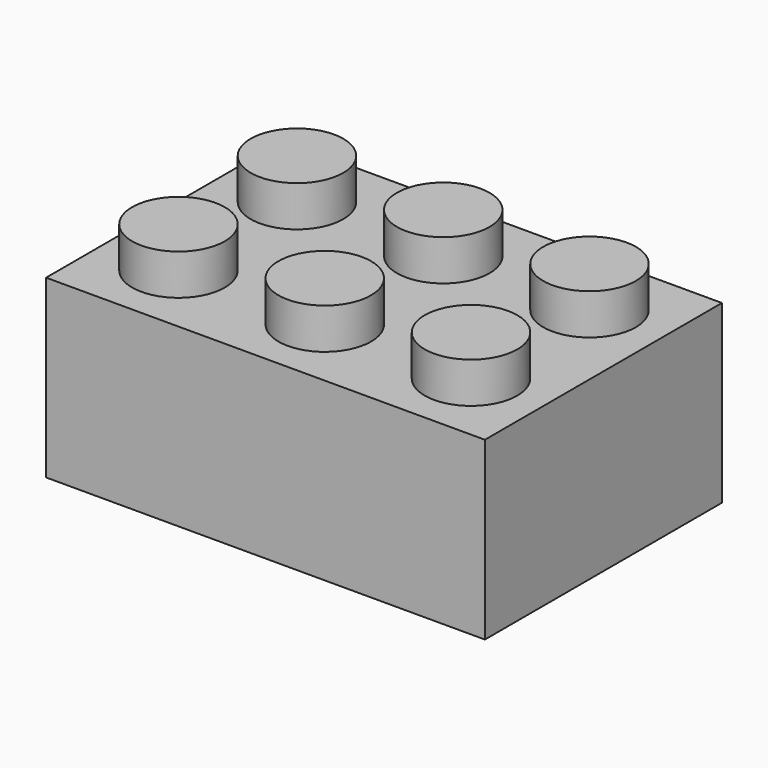
from build123d import *

# Parameters (mm, degrees)
F0_W        = 23.7
F0_H        = 8
F0_R        = 2.5
F1_DEPTH    = 9.5
F2_DEPTH    = 2.2
F4_T        = -1.5
F5_R        = 3
F6_DEPTH    = 7.9248
F7_T        = 1
F7_T3_DEPTH = 10
F7_T5_DEPTH = 15
F7_T7_DEPTH = 22.7


# Not quite as in the source:
# - a shell that OpenCascade refuses in one call is made with other operations: the cavity is built on its own and cut out


with BuildPart() as f1:
    # F0 (on Top) → F1 (new body)
    with BuildSketch(Plane.XY):
        with Locations((11.85, 4)):
            Rectangle(F0_W, F0_H)
        with Locations((3.95, 4)):
            Circle(F0_R, mode=Mode.SUBTRACT)
        with Locations((11.85, 4)):
            Circle(F0_R, mode=Mode.SUBTRACT)
        with Locations((19.75, 4)):
            Circle(F0_R, mode=Mode.SUBTRACT)
        with Locations((19.75, 4)):
            Circle(F0_R)
        with Locations((11.85, 4)):
            Circle(F0_R)
        with Locations((3.95, 4)):
            Circle(F0_R)
    extrude(amount=-F1_DEPTH)

    # F0 (on Top) → F2 (join)
    with BuildSketch(Plane.XY):
        with Locations((3.95, 4)):
            Circle(F0_R)
        with Locations((11.85, 4)):
            Circle(F0_R)
        with Locations((19.75, 4)):
            Circle(F0_R)
    extrude(amount=F2_DEPTH)

    # F3: F1 across face


with BuildPart() as f1_1:
    add(f1.part)
    add(f1.part.mirror(Plane(origin=(11.85, 0, -4.75), x_dir=(1, 0, 0), z_dir=(0, -1, 0))))

    # F4
    f4_openings = [f1_1.faces().sort_by_distance(p)[0] for p in [
        (11.85, 0, -9.5),
    ]]
    offset(amount=F4_T, openings=f4_openings, kind=Kind.INTERSECTION)

    # F5 (on face) → F6 (join)
    with BuildSketch(Plane(origin=(0, 0, -1.5), x_dir=(1, 0, 0), z_dir=(0, 0, -1))):
        with Locations((8.3, 0)):
            Circle(F5_R)
        with Locations((15.4, 0)):
            Circle(F5_R)
    extrude(amount=F6_DEPTH)

    # F7: shell of thickness 1, made by hand


with BuildPart() as f7_core1:
    # F7_t2: copy of F1
    add(f1_1.part)

    # the walls: a layer under each face that stays
    f7_faces = [f7_core1.faces().sort_by_distance(p)[0] for p in [
        (0, 0, -4.75),
        (11.85, 8, -4.75),
        (1.6928571429, -6.8571428571, -9.5),
        (11.85, -8, -4.75),
        (11.85, 0, 0),
        (23.7, 0, -4.75),
        (1.5, 0, -5.5),
        (11.85, 6.5, -5.5),
        (22.2, 0, -5.5),
        (11.85, -6.5, -5.5),
        (1.45, 4, 1.1),
        (9.35, 4, 1.1),
        (17.25, 4, 1.1),
        (17.25, -4, 1.1),
        (1.45, -4, 1.1),
        (9.35, -4, 1.1),
        (11.85, 0, -1.5),
        (3.95, 4, 2.2),
        (11.85, 4, 2.2),
        (19.75, 4, 2.2),
        (19.75, -4, 2.2),
        (3.95, -4, 2.2),
        (11.85, -4, 2.2),
        (2.95, -4, -0.4),
        (10.85, -4, -0.4),
        (18.75, -4, -0.4),
        (5.3, 0, -5.4624),
        (2.95, 4, -0.4),
        (12.4, 0, -5.4624),
        (10.85, 4, -0.4),
        (18.75, 4, -0.4),
        (3.95, -4, 0.7),
        (11.85, -4, 0.7),
        (19.75, -4, 0.7),
        (3.95, 4, 0.7),
        (11.85, 4, 0.7),
        (19.75, 4, 0.7),
    ]]
    thicken(f7_faces, amount=-F7_T, mode=Mode.SUBTRACT)

    # F7_s4 → F7_t3 (cut)
    with BuildSketch(Plane.XY.offset(-10.5)):
        Polygon((1.51, 6.49), (0.5, 6.5), (0.5, 7.5), (1.5, 7.5), align=None)
        Polygon((1.51, -6.49), (0.5, -6.5), (0.5, -7.5), (1.5, -7.5), align=None)
        Polygon((22.19, 6.49), (22.2, 7.5), (23.2, 7.5), (23.2, 6.5), align=None)
        Polygon((22.19, -6.49), (23.2, -6.5), (23.2, -7.5), (22.2, -7.5), align=None)
    extrude(amount=F7_T3_DEPTH, mode=Mode.SUBTRACT)

    # F7_s6 → F7_t5 (cut)
    with BuildSketch(Plane.XZ.offset(-7.5)):
        Polygon((1.51, -1.51), (0.5, -1.5), (0.5, -0.5), (1.5, -0.5), align=None)
        Polygon((22.19, -1.51), (23.2, -1.5), (23.2, -0.5), (22.2, -0.5), align=None)
    extrude(amount=F7_T5_DEPTH, mode=Mode.SUBTRACT)

    # F7_s8 → F7_t7 (cut)
    with BuildSketch(Plane.YZ.offset(0.5)):
        Polygon((6.49, -1.51), (7.5, -1.5), (7.5, -0.5), (6.5, -0.5), align=None)
        Polygon((-6.49, -1.51), (-7.5, -1.5), (-7.5, -0.5), (-6.5, -0.5), align=None)
    extrude(amount=F7_T7_DEPTH, mode=Mode.SUBTRACT)

    # F7_s9 → F7_t10 (revolve, cut)
    with BuildSketch(Plane.XZ.offset(-4)):
        Polygon((6.46, 0.01), (6.45, -1), (5.45, -1), (5.45, 0), align=None)
    revolve(axis=Axis((3.95, 4, 0), (0, 0, 1)), mode=Mode.SUBTRACT)

    # F7_s11 → F7_t12 (revolve, cut)
    with BuildSketch(Plane.XZ.offset(-4)):
        Polygon((14.36, 0.01), (14.35, -1), (13.35, -1), (13.35, 0), align=None)
    revolve(axis=Axis((11.85, 4, 0), (0, 0, 1)), mode=Mode.SUBTRACT)

    # F7_s13 → F7_t14 (revolve, cut)
    with BuildSketch(Plane.XZ.offset(-4)):
        Polygon((22.26, 0.01), (22.25, -1), (21.25, -1), (21.25, 0), align=None)
    revolve(axis=Axis((19.75, 4, 0), (0, 0, 1)), mode=Mode.SUBTRACT)

    # F7_s15 → F7_t16 (revolve, cut)
    with BuildSketch(Plane.XZ.offset(4)):
        Polygon((22.26, 0.01), (22.25, -1), (21.25, -1), (21.25, 0), align=None)
    revolve(axis=Axis((19.75, -4, 0), (0, 0, -1)), mode=Mode.SUBTRACT)

    # F7_s17 → F7_t18 (revolve, cut)
    with BuildSketch(Plane.XZ.offset(4)):
        Polygon((6.46, 0.01), (6.45, -1), (5.45, -1), (5.45, 0), align=None)
    revolve(axis=Axis((3.95, -4, 0), (0, 0, -1)), mode=Mode.SUBTRACT)

    # F7_s19 → F7_t20 (revolve, cut)
    with BuildSketch(Plane.XZ.offset(4)):
        Polygon((14.36, 0.01), (14.35, -1), (13.35, -1), (13.35, 0), align=None)
    revolve(axis=Axis((11.85, -4, 0), (0, 0, -1)), mode=Mode.SUBTRACT)

    # F7_s21 → F7_t22 (revolve, cut)
    with BuildSketch(Plane.XZ):
        Polygon((11.31, -1.51), (11.3, -0.5), (10.3, -0.5), (10.3, -1.5), align=None)
    revolve(axis=Axis((8.3, 0, -1.5), (0, 0, -1)), mode=Mode.SUBTRACT)

    # F7_s23 → F7_t24 (revolve, cut)
    with BuildSketch(Plane.XZ):
        Polygon((18.41, -1.51), (18.4, -0.5), (17.4, -0.5), (17.4, -1.5), align=None)
    revolve(axis=Axis((15.4, 0, -1.5), (0, 0, -1)), mode=Mode.SUBTRACT)

    # F7_s25 → F7_t26 (revolve, cut)
    with BuildSketch(Plane.XZ.offset(4)):
        Polygon((4.94, 0.69), (5.95, 0.7), (5.95, 1.7), (4.95, 1.7), align=None)
    revolve(axis=Axis((3.95, -4, 0.7), (0, 0, -1)), mode=Mode.SUBTRACT)

    # F7_s27 → F7_t28 (revolve, cut)
    with BuildSketch(Plane.XZ.offset(4)):
        Polygon((12.84, 0.69), (13.85, 0.7), (13.85, 1.7), (12.85, 1.7), align=None)
    revolve(axis=Axis((11.85, -4, 0.7), (0, 0, -1)), mode=Mode.SUBTRACT)

    # F7_s29 → F7_t30 (revolve, cut)
    with BuildSketch(Plane.XZ.offset(4)):
        Polygon((20.74, 0.69), (21.75, 0.7), (21.75, 1.7), (20.75, 1.7), align=None)
    revolve(axis=Axis((19.75, -4, 0.7), (0, 0, -1)), mode=Mode.SUBTRACT)

    # F7_s31 → F7_t32 (revolve, cut)
    with BuildSketch(Plane.XZ.offset(-4)):
        Polygon((4.94, 0.69), (5.95, 0.7), (5.95, 1.7), (4.95, 1.7), align=None)
    revolve(axis=Axis((3.95, 4, 0.7), (0, 0, -1)), mode=Mode.SUBTRACT)

    # F7_s33 → F7_t34 (revolve, cut)
    with BuildSketch(Plane.XZ.offset(-4)):
        Polygon((12.84, 0.69), (13.85, 0.7), (13.85, 1.7), (12.85, 1.7), align=None)
    revolve(axis=Axis((11.85, 4, 0.7), (0, 0, -1)), mode=Mode.SUBTRACT)

    # F7_s35 → F7_t36 (revolve, cut)
    with BuildSketch(Plane.XZ.offset(-4)):
        Polygon((20.74, 0.69), (21.75, 0.7), (21.75, 1.7), (20.75, 1.7), align=None)
    revolve(axis=Axis((19.75, 4, 0.7), (0, 0, -1)), mode=Mode.SUBTRACT)


with BuildPart() as f1_2:
    add(f1_1.part)

    # what is left inside the walls is the cavity
    f7_cavity = [f7_core1.part.solids().sort_by_distance(p)[0] for p in [
        (13.41, 0, -3.808267),
        (6.31, 0, -3.808267),
    ]]
    add(f7_cavity, mode=Mode.SUBTRACT)


solid = f1_2.part
